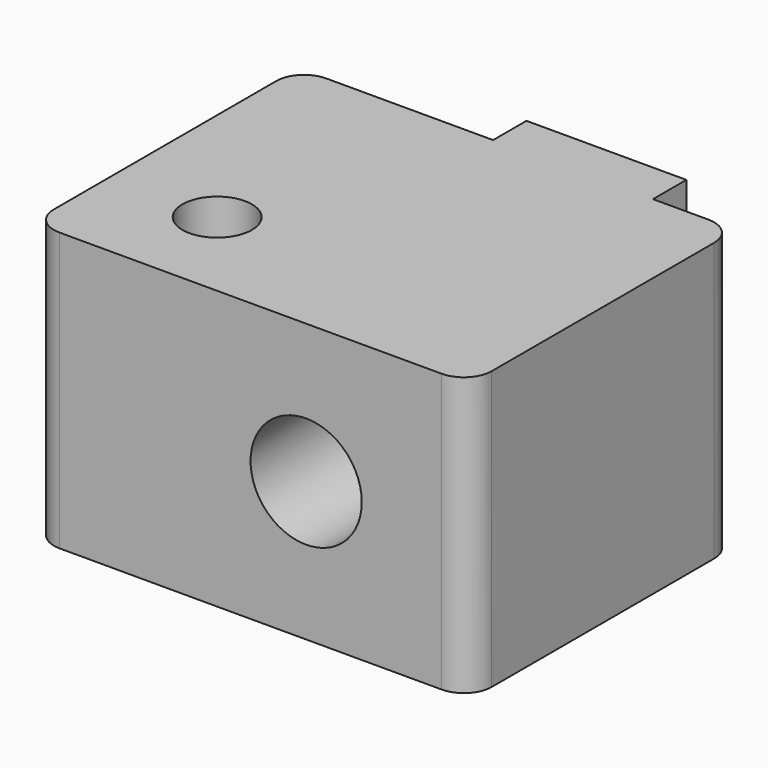
from build123d import *

# Parameters (mm, degrees)
F0_R     = 1.25
F1_DEPTH = 10
F2_R     = 2
F3_DEPTH = 13.501
F4_R     = 1


# Not quite as in the source:
# - a feature names something its author has since deleted; it is built from what else it names


with BuildPart() as f1:
    # F0 (on Top) → F1 (new body)
    with BuildSketch(Plane.XY):
        Polygon((2.875, 0), (-2.875, 0), (-2.875, -1.5), (-9.875, -1.5), (-9.875, -13.5), (5.875, -13.5), (5.875, -1.5), (2.875, -1.5), align=None)
        with Locations((-6, -10)):
            Circle(F0_R, mode=Mode.SUBTRACT)
    extrude(amount=F1_DEPTH)

    # F2 (on face) → F3 (cut, through all)
    with BuildSketch(Plane.XZ.offset(13.5)):
        with Locations((0, 5)):
            Circle(F2_R)
    extrude(amount=-F3_DEPTH, mode=Mode.SUBTRACT)

    # F4
    f4_edges = [f1.edges().sort_by_distance(p)[0] for p in [
        (5.875, -1.5, 5),
        (5.875, -13.5, 5),
        (-9.875, -1.5, 5),
        (-9.875, -13.5, 5),
    ]]
    fillet(f4_edges, radius=F4_R)


solid = f1.part
